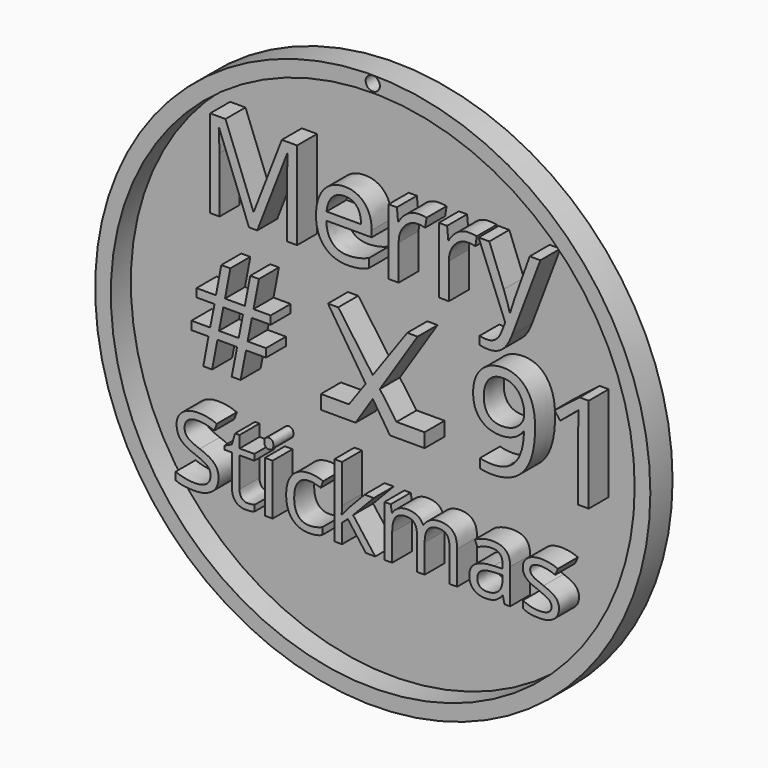
from build123d import *

# Parameters (mm, degrees)
F0_R           = 25.4
F1_DEPTH       = 2.54
F2_R           = 23.9665209366
F3_DEPTH       = 2.286
F4_TEXT_SIZE   = 11.2521125832
F4_TEXT_SIZE_2 = 8.7203858938
F5_DEPTH       = 2.286
F6_TEXT_SIZE   = 12.1708333333
F7_DEPTH       = 2.286
F8_R           = 0.650331826
F9_DEPTH       = 2.541


# Not quite as in the source:
# - Text() gives the source's letters only with a copy of the font that has no kerning and outlines rounded to 1/6400 em; it was checked with that copy


with BuildPart() as f1:
    # F0 (on Front) → F1 (new body)
    with BuildSketch(Plane.XZ):
        Circle(F0_R)
    extrude(amount=F1_DEPTH)

    # F2 (on face) → F3 (cut)
    with BuildSketch(Plane.XZ.offset(2.54)):
        Circle(F2_R)
    extrude(amount=-F3_DEPTH, mode=Mode.SUBTRACT)

    # F4 (on face) → F5 (join, through all)
    with BuildSketch(Plane.XZ.offset(0.254)):
        Polygon((-3.1558899209, 5.6634554639), (-4.1010673158, 5.6634554639), (-0.6477719242, 0.3190695634), (-2.1776105277, -1.8304506084), (-4.7430917621, -1.8304506084), (-4.7430917621, -3.113191342), (-1.5699965879, -3.113191342), (0, -0.683434638), (1.5699965879, -3.113191342), (4.7430917621, -3.113191342), (4.7430917621, -1.8304506084), (2.1776105277, -1.8304506084), (0.6477719242, 0.3190695634), (4.1010673158, 5.6634554639), (3.1558899209, 5.6634554639), (0, 1.2292301611), align=None)
        with Locations((-15.983295365, 9.4441649271)):
            Text('Merry', F4_TEXT_SIZE, font='Open Sans', text_align=(TextAlign.LEFT, TextAlign.BOTTOM))
        with Locations((-18.4812657535, -13.3076040074)):
            Text('Stickmas', F4_TEXT_SIZE_2, font='Open Sans', text_align=(TextAlign.LEFT, TextAlign.BOTTOM))
    extrude(amount=F5_DEPTH)

    # F6 (on face) → F7 (join, through all)
    with BuildSketch(Plane.XZ.offset(0.254)):
        with Locations((-16.8901125954, -3.0995445361)):
            Text('#', F6_TEXT_SIZE, font='Open Sans', text_align=(TextAlign.LEFT, TextAlign.BOTTOM))
        with Locations((8.5530917621, -3.0995445361)):
            Text('91', F6_TEXT_SIZE, font='Open Sans', text_align=(TextAlign.LEFT, TextAlign.BOTTOM))
    extrude(amount=F7_DEPTH)

    # F8 (on face) → F9 (cut, through all)
    with BuildSketch(Plane.XZ.offset(2.54)):
        with Locations((0, 24.72759597)):
            Circle(F8_R)
    extrude(amount=-F9_DEPTH, mode=Mode.SUBTRACT)


solid = f1.part
